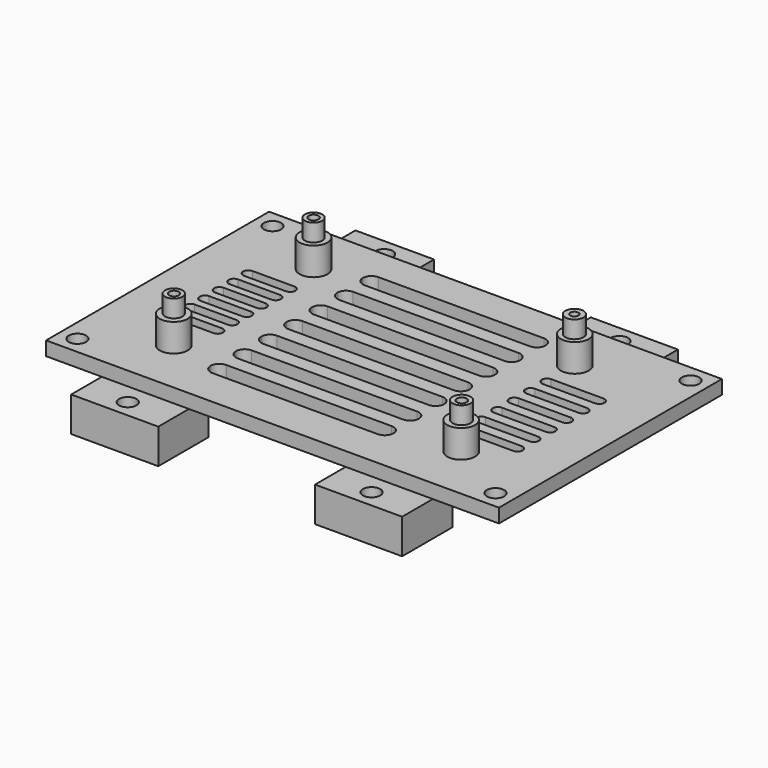
from build123d import *

# Parameters (mm, degrees)
F0_R      = 4
F1_DEPTH  = 12
F2_R      = 2.5
F3_DEPTH  = 5
F2_R_2    = 2.5937791723
F0_W      = 130
F0_H      = 80
F0_R_2    = 2.5
F4_DEPTH  = 4
F5_R      = 1.3887584209
F6_DEPTH  = 15
F5_R_2    = 1.4048695288
F7_DEPTH  = 15
F5_R_3    = 1.1639731498
F8_DEPTH  = 15
F5_R_4    = 1.43948122
F9_DEPTH  = 15
F10_W     = 25
F10_H     = 18
F10_R     = 2.5
F10_W_2   = 22.5611000657
F11_DEPTH = 10


with BuildPart() as f1:
    # F0 (on Top) → F1 (new body)
    with BuildSketch(Plane.XY):
        with Locations((25.18, 64.5)):
            Circle(F0_R)
    extrude(amount=F1_DEPTH)


with BuildPart() as f1b:
    # F0 (on Top) → F1, piece 2 (new body)
    with BuildSketch(Plane.XY):
        with Locations((100.18, 64.5)):
            Circle(F0_R)
    extrude(amount=F1_DEPTH)


with BuildPart() as f1c:
    # F0 (on Top) → F1, piece 3 (new body)
    with BuildSketch(Plane.XY):
        with Locations((106.35, 16)):
            Circle(F0_R)
    extrude(amount=F1_DEPTH)


with BuildPart() as f1d:
    # F0 (on Top) → F1, piece 4 (new body)
    with BuildSketch(Plane.XY):
        with Locations((23.85, 16)):
            Circle(F0_R)
    extrude(amount=F1_DEPTH)


with BuildPart() as f3:
    # F2 (on face) → F3 (new body)
    with BuildSketch(Plane.XY.offset(12)):
        with Locations((25.18, 64.5)):
            Circle(F2_R)
    extrude(amount=F3_DEPTH)

    # F5 (on face) → F7 (cut)
    with BuildSketch(Plane.XY.offset(17)):
        with Locations((25.18, 64.5)):
            Circle(F5_R_2)
    extrude(amount=-F7_DEPTH, mode=Mode.SUBTRACT)


with BuildPart() as f3b:
    # F2 (on face) → F3, piece 2 (new body)
    with BuildSketch(Plane.XY.offset(12)):
        with Locations((23.734146182, 16.148734875)):
            Circle(F2_R)
    extrude(amount=F3_DEPTH)

    # F5 (on face) → F6 (cut)
    with BuildSketch(Plane.XY.offset(17)):
        with Locations((23.7929187715, 16.1565169692)):
            Circle(F5_R)
    extrude(amount=-F6_DEPTH, mode=Mode.SUBTRACT)


with BuildPart() as f3c:
    # F2 (on face) → F3, piece 3 (new body)
    with BuildSketch(Plane.XY.offset(12)):
        with Locations((100.1164472483, 64.4212665508)):
            Circle(F2_R_2)
    extrude(amount=F3_DEPTH)

    # F5 (on face) → F8 (cut)
    with BuildSketch(Plane.XY.offset(17)):
        with Locations((100.1068949699, 64.436905086)):
            Circle(F5_R_3)
    extrude(amount=-F8_DEPTH, mode=Mode.SUBTRACT)


with BuildPart() as f3d:
    # F2 (on face) → F3, piece 4 (new body)
    with BuildSketch(Plane.XY.offset(12)):
        with Locations((106.4064774143, 16.0643732485)):
            Circle(F2_R_2)
    extrude(amount=F3_DEPTH)

    # F5 (on face) → F9 (cut)
    with BuildSketch(Plane.XY.offset(17)):
        with Locations((106.5456867218, 15.9565918148)):
            Circle(F5_R_4)
    extrude(amount=-F9_DEPTH, mode=Mode.SUBTRACT)


with BuildPart() as f4:
    # F0 (on Top) → F4 (new body)
    with BuildSketch(Plane.XY):
        with Locations((65, 40)):
            Rectangle(F0_W, F0_H)
        with Locations((5, 5)):
            Circle(F0_R_2, mode=Mode.SUBTRACT)
        with Locations((23.85, 16)):
            Circle(F0_R, mode=Mode.SUBTRACT)
        with BuildLine():
            Line((86.5, 10.9), (39, 10.9))
            ThreePointArc((39, 10.9), (37.232233047, 11.632233047), (36.5, 13.4))
            ThreePointArc((36.5, 13.4), (37.232233047, 15.167766953), (39, 15.9))
            Line((39, 15.9), (86.5, 15.9))
            ThreePointArc((86.5, 15.9), (88.267766953, 15.167766953), (89, 13.4))
            ThreePointArc((89, 13.4), (88.267766953, 11.632233047), (86.5, 10.9))
        make_face(mode=Mode.SUBTRACT)
        with BuildLine():
            ThreePointArc((13.5966599469, 27.7040311471), (14.0359997751, 28.7646913189), (15.0966599469, 29.2040311471))
            Line((15.0966599469, 29.2040311471), (27.0966599469, 29.2040311471))
            ThreePointArc((27.0966599469, 29.2040311471), (28.1573201187, 28.7646913189), (28.5966599469, 27.7040311471))
            ThreePointArc((28.5966599469, 27.7040311471), (28.1573201187, 26.6433709754), (27.0966599469, 26.2040311471))
            Line((27.0966599469, 26.2040311471), (15.0966599469, 26.2040311471))
            ThreePointArc((15.0966599469, 26.2040311471), (14.0359997751, 26.6433709754), (13.5966599469, 27.7040311471))
        make_face(mode=Mode.SUBTRACT)
        with BuildLine():
            ThreePointArc((13.597495122, 32.9040310801), (14.0368349503, 33.9646912518), (15.097495122, 34.4040310801))
            Line((15.097495122, 34.4040310801), (27.097495122, 34.4040310801))
            ThreePointArc((27.097495122, 34.4040310801), (28.1581552938, 33.9646912518), (28.597495122, 32.9040310801))
            ThreePointArc((28.597495122, 32.9040310801), (28.1581552938, 31.8433709083), (27.097495122, 31.4040310801))
            Line((27.097495122, 31.4040310801), (15.097495122, 31.4040310801))
            ThreePointArc((15.097495122, 31.4040310801), (14.0368349503, 31.8433709083), (13.597495122, 32.9040310801))
        make_face(mode=Mode.SUBTRACT)
        with BuildLine():
            ThreePointArc((13.5983302972, 38.104031013), (14.0376701254, 39.1646911848), (15.0983302972, 39.604031013))
            Line((15.0983302972, 39.604031013), (27.0983302972, 39.604031013))
            ThreePointArc((27.0983302972, 39.604031013), (28.1589904689, 39.1646911848), (28.5983302972, 38.104031013))
            ThreePointArc((28.5983302972, 38.104031013), (28.1589904689, 37.0433708412), (27.0983302972, 36.604031013))
            Line((27.0983302972, 36.604031013), (15.0983302972, 36.604031013))
            ThreePointArc((15.0983302972, 36.604031013), (14.0376701254, 37.0433708412), (13.5983302972, 38.104031013))
        make_face(mode=Mode.SUBTRACT)
        with BuildLine():
            Line((86.5, 20), (39, 20))
            ThreePointArc((39, 20), (37.232233047, 20.732233047), (36.5, 22.5))
            ThreePointArc((36.5, 22.5), (37.232233047, 24.267766953), (39, 25))
            Line((39, 25), (86.5, 25))
            ThreePointArc((86.5, 25), (88.267766953, 24.267766953), (89, 22.5))
            ThreePointArc((89, 22.5), (88.267766953, 20.732233047), (86.5, 20))
        make_face(mode=Mode.SUBTRACT)
        with BuildLine():
            Line((86.5, 29.1), (39, 29.1))
            ThreePointArc((39, 29.1), (37.232233047, 29.832233047), (36.5, 31.6))
            ThreePointArc((36.5, 31.6), (37.232233047, 33.367766953), (39, 34.1))
            Line((39, 34.1), (86.5, 34.1))
            ThreePointArc((86.5, 34.1), (88.267766953, 33.367766953), (89, 31.6))
            ThreePointArc((89, 31.6), (88.267766953, 29.832233047), (86.5, 29.1))
        make_face(mode=Mode.SUBTRACT)
        with Locations((125, 5)):
            Circle(F0_R_2, mode=Mode.SUBTRACT)
        with Locations((106.35, 16)):
            Circle(F0_R, mode=Mode.SUBTRACT)
        with BuildLine():
            ThreePointArc((98.7730469401, 25.0220314212), (99.2123867683, 26.0826915929), (100.2730469401, 26.5220314212))
            Line((100.2730469401, 26.5220314212), (115.2730469401, 26.5220314212))
            ThreePointArc((115.2730469401, 26.5220314212), (116.3337071119, 26.0826915929), (116.7730469401, 25.0220314212))
            ThreePointArc((116.7730469401, 25.0220314212), (116.3337071119, 23.9613712494), (115.2730469401, 23.5220314212))
            Line((115.2730469401, 23.5220314212), (100.2730469401, 23.5220314212))
            ThreePointArc((100.2730469401, 23.5220314212), (99.2123867683, 23.9613712494), (98.7730469401, 25.0220314212))
        make_face(mode=Mode.SUBTRACT)
        with BuildLine():
            ThreePointArc((98.7549219724, 30.9220035809), (99.1942618006, 31.9826637527), (100.2549219724, 32.4220035809))
            Line((100.2549219724, 32.4220035809), (115.2549219724, 32.4220035809))
            ThreePointArc((115.2549219724, 32.4220035809), (116.3155821442, 31.9826637527), (116.7549219724, 30.9220035809))
            ThreePointArc((116.7549219724, 30.9220035809), (116.3155821442, 29.8613434091), (115.2549219724, 29.4220035809))
            Line((115.2549219724, 29.4220035809), (100.2549219724, 29.4220035809))
            ThreePointArc((100.2549219724, 29.4220035809), (99.1942618006, 29.8613434091), (98.7549219724, 30.9220035809))
        make_face(mode=Mode.SUBTRACT)
        with BuildLine():
            ThreePointArc((98.7367970047, 36.8219757406), (99.1761368329, 37.8826359124), (100.2367970047, 38.3219757406))
            Line((100.2367970047, 38.3219757406), (115.2367970047, 38.3219757406))
            ThreePointArc((115.2367970047, 38.3219757406), (116.2974571764, 37.8826359124), (116.7367970047, 36.8219757406))
            ThreePointArc((116.7367970047, 36.8219757406), (116.2974571764, 35.7613155688), (115.2367970047, 35.3219757406))
            Line((115.2367970047, 35.3219757406), (100.2367970047, 35.3219757406))
            ThreePointArc((100.2367970047, 35.3219757406), (99.1761368329, 35.7613155688), (98.7367970047, 36.8219757406))
        make_face(mode=Mode.SUBTRACT)
        with BuildLine():
            ThreePointArc((13.5991654723, 43.3040309459), (14.0385053005, 44.3646911177), (15.0991654723, 44.8040309459))
            Line((15.0991654723, 44.8040309459), (27.0991654723, 44.8040309459))
            ThreePointArc((27.0991654723, 44.8040309459), (28.1598256441, 44.3646911177), (28.5991654723, 43.3040309459))
            ThreePointArc((28.5991654723, 43.3040309459), (28.1598256441, 42.2433707741), (27.0991654723, 41.8040309459))
            Line((27.0991654723, 41.8040309459), (15.0991654723, 41.8040309459))
            ThreePointArc((15.0991654723, 41.8040309459), (14.0385053005, 42.2433707741), (13.5991654723, 43.3040309459))
        make_face(mode=Mode.SUBTRACT)
        with BuildLine():
            ThreePointArc((13.6000006474, 48.5040308789), (14.0393404756, 49.5646910506), (15.1000006474, 50.0040308789))
            Line((15.1000006474, 50.0040308789), (27.1000006474, 50.0040308789))
            ThreePointArc((27.1000006474, 50.0040308789), (28.1606608192, 49.5646910506), (28.6000006474, 48.5040308789))
            ThreePointArc((28.6000006474, 48.5040308789), (28.1606608192, 47.4433707071), (27.1000006474, 47.0040308789))
            Line((27.1000006474, 47.0040308789), (15.1000006474, 47.0040308789))
            ThreePointArc((15.1000006474, 47.0040308789), (14.0393404756, 47.4433707071), (13.6000006474, 48.5040308789))
        make_face(mode=Mode.SUBTRACT)
        with BuildLine():
            ThreePointArc((13.6008358225, 53.7040308118), (14.0401756507, 54.7646909836), (15.1008358225, 55.2040308118))
            Line((15.1008358225, 55.2040308118), (27.1008358225, 55.2040308118))
            ThreePointArc((27.1008358225, 55.2040308118), (28.1614959943, 54.7646909836), (28.6008358225, 53.7040308118))
            ThreePointArc((28.6008358225, 53.7040308118), (28.1614959943, 52.64337064), (27.1008358225, 52.2040308118))
            Line((27.1008358225, 52.2040308118), (15.1008358225, 52.2040308118))
            ThreePointArc((15.1008358225, 52.2040308118), (14.0401756507, 52.64337064), (13.6008358225, 53.7040308118))
        make_face(mode=Mode.SUBTRACT)
        with BuildLine():
            Line((86.5, 38.2), (39, 38.2))
            ThreePointArc((39, 38.2), (37.232233047, 38.932233047), (36.5, 40.7))
            ThreePointArc((36.5, 40.7), (37.232233047, 42.467766953), (39, 43.2))
            Line((39, 43.2), (86.5, 43.2))
            ThreePointArc((86.5, 43.2), (88.267766953, 42.467766953), (89, 40.7))
            ThreePointArc((89, 40.7), (88.267766953, 38.932233047), (86.5, 38.2))
        make_face(mode=Mode.SUBTRACT)
        with BuildLine():
            Line((86.5, 47.3), (39, 47.3))
            ThreePointArc((39, 47.3), (37.232233047, 48.032233047), (36.5, 49.8))
            ThreePointArc((36.5, 49.8), (37.232233047, 51.567766953), (39, 52.3))
            Line((39, 52.3), (86.5, 52.3))
            ThreePointArc((86.5, 52.3), (88.267766953, 51.567766953), (89, 49.8))
            ThreePointArc((89, 49.8), (88.267766953, 48.032233047), (86.5, 47.3))
        make_face(mode=Mode.SUBTRACT)
        with BuildLine():
            Line((86.5, 56.4), (39, 56.4))
            ThreePointArc((39, 56.4), (37.232233047, 57.132233047), (36.5, 58.9))
            ThreePointArc((36.5, 58.9), (37.232233047, 60.667766953), (39, 61.4))
            Line((39, 61.4), (86.5, 61.4))
            ThreePointArc((86.5, 61.4), (88.267766953, 60.667766953), (89, 58.9))
            ThreePointArc((89, 58.9), (88.267766953, 57.132233047), (86.5, 56.4))
        make_face(mode=Mode.SUBTRACT)
        with Locations((25.18, 64.5)):
            Circle(F0_R, mode=Mode.SUBTRACT)
        with Locations((5, 75)):
            Circle(F0_R_2, mode=Mode.SUBTRACT)
        with BuildLine():
            ThreePointArc((36.5, 68), (37.232233047, 69.767766953), (39, 70.5))
            Line((39, 70.5), (86.5, 70.5))
            ThreePointArc((86.5, 70.5), (88.267766953, 69.767766953), (89, 68))
            ThreePointArc((89, 68), (88.267766953, 66.232233047), (86.5, 65.5))
            Line((86.5, 65.5), (39, 65.5))
            ThreePointArc((39, 65.5), (37.232233047, 66.232233047), (36.5, 68))
        make_face(mode=Mode.SUBTRACT)
        with BuildLine():
            ThreePointArc((98.7186720369, 42.7219479003), (99.1580118652, 43.7826080721), (100.2186720369, 44.2219479003))
            Line((100.2186720369, 44.2219479003), (115.2186720369, 44.2219479003))
            ThreePointArc((115.2186720369, 44.2219479003), (116.2793322087, 43.7826080721), (116.7186720369, 42.7219479003))
            ThreePointArc((116.7186720369, 42.7219479003), (116.2793322087, 41.6612877285), (115.2186720369, 41.2219479003))
            Line((115.2186720369, 41.2219479003), (100.2186720369, 41.2219479003))
            ThreePointArc((100.2186720369, 41.2219479003), (99.1580118652, 41.6612877285), (98.7186720369, 42.7219479003))
        make_face(mode=Mode.SUBTRACT)
        with BuildLine():
            ThreePointArc((98.7005470692, 48.6219200601), (99.1398868974, 49.6825802318), (100.2005470692, 50.1219200601))
            Line((100.2005470692, 50.1219200601), (115.2005470692, 50.1219200601))
            ThreePointArc((115.2005470692, 50.1219200601), (116.261207241, 49.6825802318), (116.7005470692, 48.6219200601))
            ThreePointArc((116.7005470692, 48.6219200601), (116.261207241, 47.5612598883), (115.2005470692, 47.1219200601))
            Line((115.2005470692, 47.1219200601), (100.2005470692, 47.1219200601))
            ThreePointArc((100.2005470692, 47.1219200601), (99.1398868974, 47.5612598883), (98.7005470692, 48.6219200601))
        make_face(mode=Mode.SUBTRACT)
        with BuildLine():
            ThreePointArc((98.6824221015, 54.5218922198), (99.1217619297, 55.5825523916), (100.1824221015, 56.0218922198))
            Line((100.1824221015, 56.0218922198), (115.1824221015, 56.0218922198))
            ThreePointArc((115.1824221015, 56.0218922198), (116.2430822733, 55.5825523916), (116.6824221015, 54.5218922198))
            ThreePointArc((116.6824221015, 54.5218922198), (116.2430822733, 53.461232048), (115.1824221015, 53.0218922198))
            Line((115.1824221015, 53.0218922198), (100.1824221015, 53.0218922198))
            ThreePointArc((100.1824221015, 53.0218922198), (99.1217619297, 53.461232048), (98.6824221015, 54.5218922198))
        make_face(mode=Mode.SUBTRACT)
        with Locations((100.18, 64.5)):
            Circle(F0_R, mode=Mode.SUBTRACT)
        with Locations((125, 75)):
            Circle(F0_R_2, mode=Mode.SUBTRACT)
    extrude(amount=F4_DEPTH)

    # F10 (on face) → F11 (join)
    with BuildSketch(Plane.XY):
        with Locations((28.5, -2)):
            Rectangle(F10_W, F10_H)
        with Locations((28.23, -6)):
            Circle(F10_R, mode=Mode.SUBTRACT)
        with Locations((98.5, -2)):
            Rectangle(F10_W, F10_H)
        with Locations((98.23, -6)):
            Circle(F10_R, mode=Mode.SUBTRACT)
        with Locations((27.2805500329, 82)):
            Rectangle(F10_W_2, F10_H)
        with Locations((28.23, 86)):
            Circle(F10_R, mode=Mode.SUBTRACT)
        with Locations((96.0611000657, 82)):
            Rectangle(F10_W, F10_H)
        with Locations((95.7911000657, 86)):
            Circle(F10_R, mode=Mode.SUBTRACT)
    extrude(amount=-F11_DEPTH)


solid = Compound([f1.part, f1b.part, f1c.part, f1d.part, f3.part, f3b.part, f3c.part, f3d.part, f4.part])
